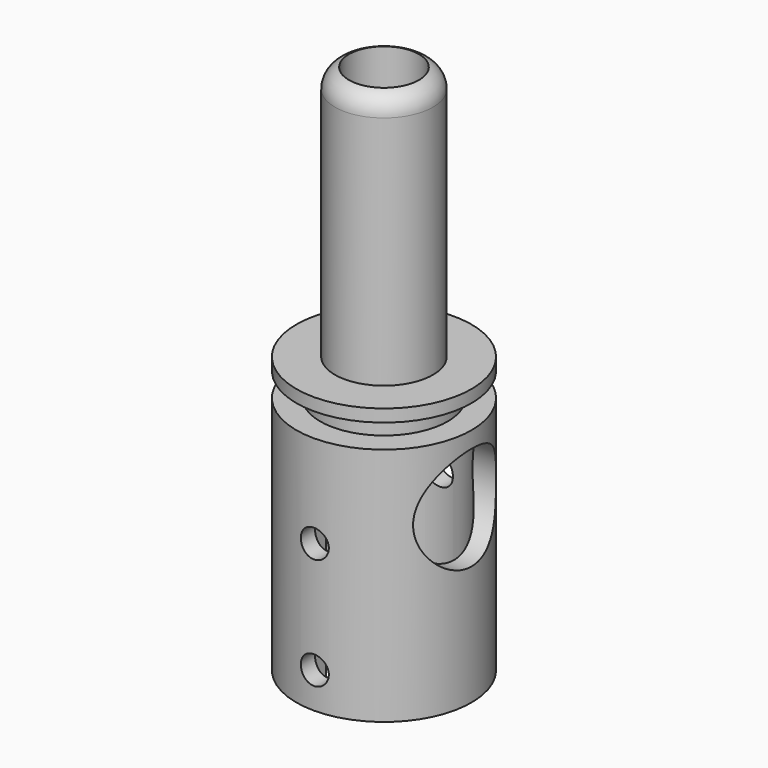
from build123d import *

# Parameters (mm, degrees)
F5_D      = 7.4
F5_DEPTH  = 2
F5_START  = 2.3628878
F5_TIP    = 2.2231842904
F8_D      = 2
F10_W     = 1.5
F10_H     = 1.7
F11_DEPTH = 1.8
F13_W     = 1.5
F13_H     = 1.5
F14_DEPTH = 12.9


# Not quite as in the source:
# - a fillet or chamfer that OpenCascade refuses, or shapes differently, is made with other operations: its cross-section is extruded or revolved along the edge and cut away or added


with BuildPart() as f1:
    # F0 (on Right) → F1 (revolve)
    with BuildSketch(Plane.YZ):
        Polygon((-2.5, 27.272233048), (-3.5, 27.272233048), (-3.5, 9.072233048), (-6.25, 9.072233048), (-6.25, 8.1851361653), (-4.55, 8.1851361653), (-4.55, 6.4851361653), (-6.25, 6.4851361653), (-6.25, 5.042233048), (-6.25, -10.627766952), (-5, -10.627766952), (-5, 5.042233048), (-2.5, 7.3351361653), align=None)
    revolve(axis=Axis((0, 0, 6.4422870055), (0, 0, -1)))

    # F2: fillet of radius 1.4485281374 on 1 edges, made by hand

    # F2_s1 → F2_t2 (revolve, cut)
    with BuildSketch(Plane.YZ):
        with BuildLine():
            ThreePointArc((-2.5, 27.272233048), (-3.2236363972, 26.7459334429), (-3.5, 25.8948963881))
            Line((-3.5, 25.8948963881), (-3.5, 27.272233048))
            Line((-3.5, 27.272233048), (-2.5, 27.272233048))
        make_face()
    revolve(axis=Axis((0, 0, 27.272233048), (0, 0, -1)), mode=Mode.SUBTRACT)

    # F5
    # its depths count from where the whole tool has entered the part; down to there all is cleared
    with Locations(Plane.YZ.offset(7.4)):
        with Locations((0, 1.622233048)):
            Hole(F5_D / 2, depth=F5_START)
    with Locations(Plane.YZ.offset(7.4).offset(-F5_START)):
        with Locations((0, 1.622233048)):
            Hole(F5_D / 2, depth=F5_DEPTH)
            with Locations((0, 0, -(F5_DEPTH + F5_TIP / 2))):  # 118° drill point
                Cone(0, F5_D / 2, F5_TIP, mode=Mode.SUBTRACT)

    # F8 (through all)
    with Locations(Plane.XZ.offset(7.5)):
        with Locations((0, -8.077766952), (0, -0.127766952)):
            Hole(F8_D / 2)

    # F13 (on Top) → F14 (join)
    with BuildSketch(Plane.XY):
        with Locations((-5.5, 0)):
            Rectangle(F13_W, F13_H)
    extrude(amount=-F14_DEPTH)


with BuildPart() as f11:
    # F10 (on offset) → F11 (new body)
    with BuildSketch(Plane.YZ.offset(-6.27)):
        with Locations((-0.0197449699, -11.4840940437)):
            Rectangle(F10_W, F10_H)
    extrude(amount=F11_DEPTH)


solid = f1.part
